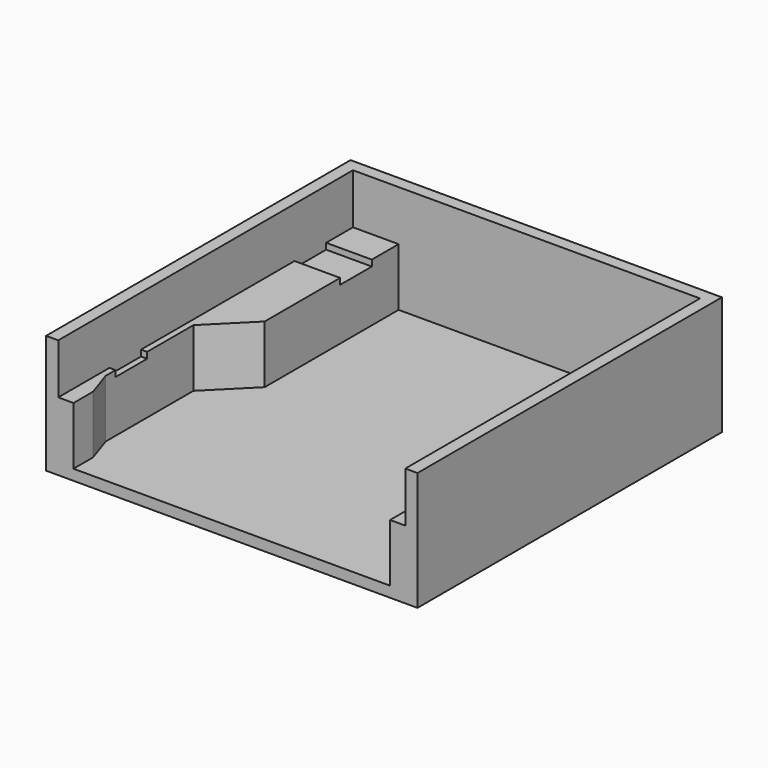
from build123d import *

# Parameters (mm, degrees)
F0_W     = 1549.4
F0_H     = 1587.5
F1_DEPTH = 495.3
F2_W     = 1447.8
F2_H     = 1536.7
F3_DEPTH = 209.55
F5_DEPTH = 241.3
F6_SIZE  = 165.09999
F7_SIZE  = 165.09999
F8_W     = 192.0828819275
F8_H     = 165.1
F8_W_2   = 25.4
F8_W_3   = 25.217294693
F8_W_4   = 190.5
F9_DEPTH = 25.4


# Not quite as in the source:
# - a fillet or chamfer is up to 0.001 mm smaller than in the source, because OpenCascade refuses the exact size


with BuildPart() as f1:
    # F0 (on Top) → F1 (new body)
    with BuildSketch(Plane.XY):
        with Locations((774.7, 793.75)):
            Rectangle(F0_W, F0_H)
    extrude(amount=F1_DEPTH)

    # F2 (on face) → F3 (cut)
    with BuildSketch(Plane.XY.offset(495.3)):
        with Locations((774.7, 768.35)):
            Rectangle(F2_W, F2_H)
    extrude(amount=-F3_DEPTH, mode=Mode.SUBTRACT)

    # F4 (on face) → F5 (cut)
    with BuildSketch(Plane.XY.offset(285.75)):
        Polygon((114.3, 101.6), (114.3, 0), (1435.1, 0), (1435.1, 101.6), (1473.2, 215.9), (1473.2, 673.1), (1308.1, 673.1), (1308.1, 1536.7), (241.3, 1536.7), (241.3, 673.1), (76.2, 673.1), (76.2, 215.9), align=None)
    extrude(amount=-F5_DEPTH, mode=Mode.SUBTRACT)

    # F6 (size 165.1 in the source; OpenCascade refuses exactly that, so slightly less here)
    f6_edges = [f1.edges().sort_by_distance(p)[0] for p in [
        (241.3, 673.1, 165.1),
    ]]
    chamfer(f6_edges, length=F6_SIZE)

    # F7 (size 165.1 in the source; OpenCascade refuses exactly that, so slightly less here)
    f7_edges = [f1.edges().sort_by_distance(p)[0] for p in [
        (1308.1, 673.1, 165.1),
    ]]
    chamfer(f7_edges, length=F7_SIZE)

    # F8 (on face) → F9 (cut)
    with BuildSketch(Plane.XY.offset(285.75)):
        with Locations((1403.493642807, 1314.45)):
            Rectangle(F8_W, F8_H)
        with Locations((63.5, 349.25)):
            Rectangle(F8_W_2, F8_H)
        with Locations((1485.9412908554, 349.25)):
            Rectangle(F8_W_3, F8_H)
        with Locations((146.05, 1314.45)):
            Rectangle(F8_W_4, F8_H)
    extrude(amount=-F9_DEPTH, mode=Mode.SUBTRACT)


solid = f1.part
